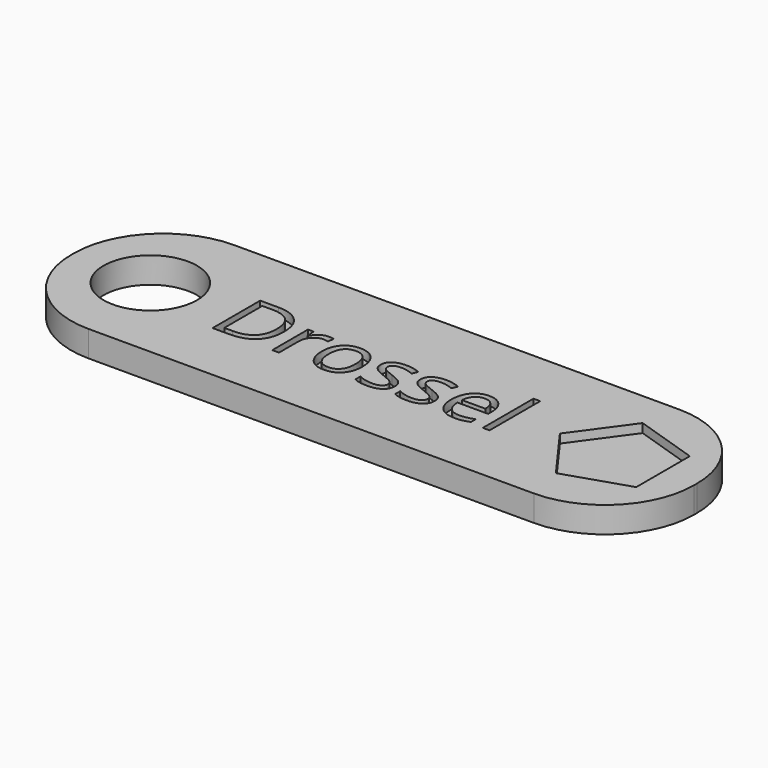
from build123d import *

# Parameters (mm, degrees)
F0_W         = 120
F0_H         = 35
F0_R         = 9
F1_DEPTH     = 5
F3_R         = 17.1409162928
F2_TEXT_SIZE = 16.0361853583
F4_DEPTH     = 1.7


# Not quite as in the source:
# - Text() gives the source's letters only with a copy of the font that has no kerning and outlines rounded to 1/6400 em; it was checked with that copy


with BuildPart() as f1:
    # F0 (on Top) → F1 (new body)
    with BuildSketch(Plane.XY):
        Rectangle(F0_W, F0_H)
        with Locations((-45, 0)):
            Circle(F0_R, mode=Mode.SUBTRACT)
    extrude(amount=F1_DEPTH)

    # F3
    f3_edges = [f1.edges().sort_by_distance(p)[0] for p in [
        (-60, -17.5, 2.5),
        (60, 17.5, 2.5),
        (-60, 17.5, 2.5),
        (60, -17.5, 2.5),
    ]]
    fillet(f3_edges, radius=F3_R)

    # F2 (on face) → F4 (cut)
    with BuildSketch(Plane.XY.offset(5)):
        Polygon((53.5880746414, -6.280463604), (53.5880746414, 6.6252222774), (41.3140379866, 10.6132985389), (33.7282661547, 0.1723793367), (41.3140379866, -10.2685398655), align=None)
        with Locations((-30.0766932778, -5.6250006892)):
            Text('Drossel', F2_TEXT_SIZE, font='Open Sans', text_align=(TextAlign.LEFT, TextAlign.BOTTOM))
    extrude(amount=-F4_DEPTH, mode=Mode.SUBTRACT)


solid = f1.part
